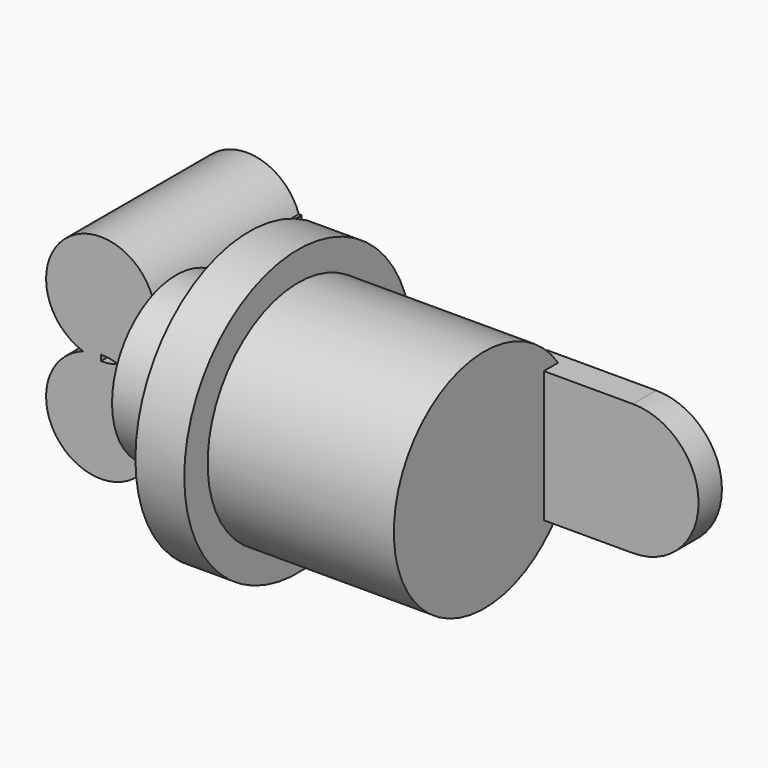
from build123d import *

# Parameters (mm, degrees)
F0_R      = 11.4211526137
F1_DEPTH  = 5.08
F3_R      = 19.685
F4_DEPTH  = 40.894
F6_DEPTH  = 5.08
F9_R      = 24.765
F10_DEPTH = 8.5
F11_R     = 13.97
F12_DEPTH = 12.7
F15_DEPTH = 31.75


with BuildPart() as f1:
    # F0 (on Front) → F1 (new body)
    with BuildSketch(Plane.XZ):
        Circle(F0_R)
    extrude(amount=F1_DEPTH)



with BuildPart() as f4:
    # F3 (on offset) → F4 (new body)
    with BuildSketch(Plane.YZ.offset(-15.5)):
        with Locations((-18, 0)):
            Circle(F3_R)
    extrude(amount=-F4_DEPTH)


with BuildPart() as f1_1:
    add(f1.part)

    add(f4.part)  # F6 merges F4
    # F5 (on face) → F6 (join, through all)
    with BuildSketch(Plane(origin=(0, 0, 0), x_dir=(-1, 0, 0), z_dir=(0, 1, 0))):
        with BuildLine():
            Line((19.05, 11.4211526137), (0, 11.4211526137))
            ThreePointArc((0, 11.4211526137), (8.0759744621, 8.0759744621), (11.4211526137, 0))
            ThreePointArc((11.4211526137, 0), (8.0759744621, -8.0759744621), (0, -11.4211526137))
            Line((0, -11.4211526137), (19.05, -11.4211526137))
            Line((19.05, -11.4211526137), (19.05, 11.4211526137))
        make_face()
    extrude(amount=-F6_DEPTH)

    # F9 (on face) → F10 (join)
    with BuildSketch(Plane(origin=(-56.394, 0, 0), x_dir=(0, -1, 0), z_dir=(-1, 0, 0))):
        with Locations((18, 0)):
            Circle(F9_R)
    extrude(amount=-F10_DEPTH)

    # F11 (on face) → F12 (join)
    with BuildSketch(Plane(origin=(-56.394, 0, 0), x_dir=(0, -1, 0), z_dir=(-1, 0, 0))):
        with Locations((18, 0)):
            Circle(F11_R)
    extrude(amount=F12_DEPTH)

    # F14 (on offset) → F15 (join)
    with BuildSketch(Plane.XZ.offset(22.5)):
        with BuildLine():
            ThreePointArc((-75.5499063227, 0), (-70.8743650094, 3.472069535), (-69.094, 9.017))
            ThreePointArc((-69.094, 9.017), (-69.2170356699, 10.5430051561), (-69.5829641441, 12.0295870961))
            Line((-69.5829641441, 12.0295870961), (-78.619, 12.0295870961))
            Line((-78.619, 12.0295870961), (-78.619, 0.508))
            ThreePointArc((-78.619, 0.508), (-77.0635740133, 0.3801418527), (-75.5499063227, 0))
        make_face()
        with BuildLine():
            Line((-69.094, -9.017), (-69.094, 9.017))
            ThreePointArc((-69.094, 9.017), (-70.8743650094, 3.472069535), (-75.5499063227, 0))
            ThreePointArc((-75.5499063227, 0), (-70.8743650094, -3.472069535), (-69.094, -9.017))
        make_face()
        with BuildLine():
            ThreePointArc((-69.5829641441, 12.0295870961), (-69.2170356699, 10.5430051561), (-69.094, 9.017))
            Line((-69.094, 9.017), (-69.094, 12.0295870961))
            Line((-69.094, 12.0295870961), (-69.5829641441, 12.0295870961))
        make_face()
        with BuildLine():
            Line((-78.619, 12.0295870961), (-69.5829641441, 12.0295870961))
            ThreePointArc((-69.5829641441, 12.0295870961), (-85.3330778344, 15.7732403624), (-81.6880936773, 0))
            ThreePointArc((-81.6880936773, 0), (-80.1744259867, 0.3801418527), (-78.619, 0.508))
            Line((-78.619, 0.508), (-78.619, 12.0295870961))
        make_face()
        with BuildLine():
            ThreePointArc((-69.094, -9.017), (-70.8743650094, -3.472069535), (-75.5499063227, 0))
            ThreePointArc((-75.5499063227, 0), (-77.0635740133, -0.3801418527), (-78.619, -0.508))
            Line((-78.619, -0.508), (-78.619, -12.0295870961))
            Line((-78.619, -12.0295870961), (-69.5829641441, -12.0295870961))
            ThreePointArc((-69.5829641441, -12.0295870961), (-69.2170356699, -10.5430051561), (-69.094, -9.017))
        make_face()
        with BuildLine():
            Line((-69.094, -12.0295870961), (-69.094, -9.017))
            ThreePointArc((-69.094, -9.017), (-69.2170356699, -10.5430051561), (-69.5829641441, -12.0295870961))
            Line((-69.5829641441, -12.0295870961), (-69.094, -12.0295870961))
        make_face()
        with BuildLine():
            ThreePointArc((-78.619, 0.508), (-80.1744259867, 0.3801418527), (-81.6880936773, 0))
            ThreePointArc((-81.6880936773, 0), (-80.1744259867, -0.3801418527), (-78.619, -0.508))
            Line((-78.619, -0.508), (-78.619, 0.508))
        make_face()
        with BuildLine():
            ThreePointArc((-78.619, -0.508), (-80.1744259867, -0.3801418527), (-81.6880936773, 0))
            ThreePointArc((-81.6880936773, 0), (-85.3330778344, -15.7732403624), (-69.5829641441, -12.0295870961))
            Line((-69.5829641441, -12.0295870961), (-78.619, -12.0295870961))
            Line((-78.619, -12.0295870961), (-78.619, -0.508))
        make_face()
    extrude(amount=-F15_DEPTH)


solid = f1_1.part
